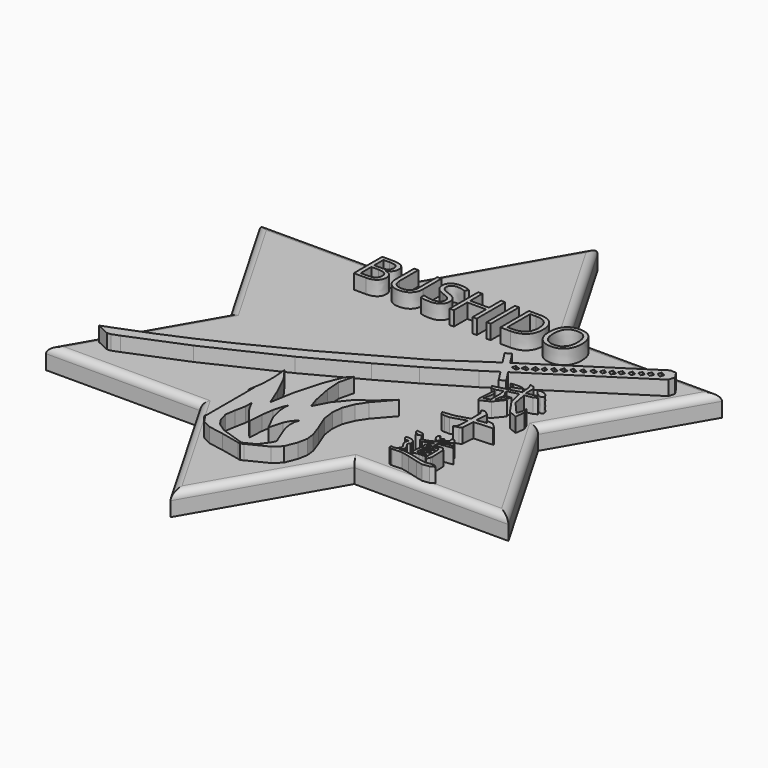
from build123d import *

# Parameters (mm, degrees)
F1_TEXT_SIZE = 8.7433378212
F5_DEPTH     = 2.54
F6_DEPTH     = 3.81
F7_R         = 1.27


# Not quite as in the source:
# - Text() gives the source's letters only with a copy of the font that has no kerning and outlines rounded to 1/6400 em; it was checked with that copy


with BuildPart() as f5:
    # F1 (on Top) + F2 (on Top) + F3 (on Top) + F4 (on Top) → F5 (new body)
    with BuildSketch(Plane.XY):
        with Locations((-18.8456885517, 15.8561766148)):
            Text('BUSHIDO', F1_TEXT_SIZE, font='Open Sans', text_align=(TextAlign.LEFT, TextAlign.BOTTOM))
    with BuildSketch(Plane.XY):
        Polygon((16.8473965077, 6.140861365), (15.3403033092, 8.4730714844), (13.8332103635, 10.8052812126), (12.9538516546, 10.2370324437), (14.4609446004, 7.9048227154), (15.9680377988, 5.5726125961), (17.3082601312, 3.4986333036), (18.2062507596, 4.0380493823), align=None)
        Polygon((33.8832835333, 20.4556965248), (15.3403033092, 8.4730714844), (16.8473965077, 6.140861365), (35.3903767318, 18.1234864055), (35.6585590299, 19.2181617838), (34.9173655604, 20.3651505113), align=None)
        Polygon((16.3403138651, 7.6048727276), (16.5452819858, 8.2522101603), (17.3955264899, 7.9045698589), (17.2131276315, 7.3285114539), align=None, mode=Mode.SUBTRACT)
        Polygon((17.5423044973, 8.2190133387), (17.6540358979, 8.9686959803), (18.5137291101, 8.6353379366), (18.4319203078, 8.0864265413), align=None, mode=Mode.SUBTRACT)
        Polygon((18.7442950032, 8.8331541453), (18.8201417398, 9.722243085), (19.6246346881, 9.4333665485), (19.567441079, 8.7629328875), align=None, mode=Mode.SUBTRACT)
        Polygon((19.880105257, 9.6755209268), (19.909781471, 10.4263771654), (20.5806503807, 10.1011195962), (20.5139143984, 9.4076129406), align=None, mode=Mode.SUBTRACT)
        Polygon((20.9012147802, 10.4437671608), (21.0185353832, 11.1428629854), (21.9333342245, 10.6891891454), (21.6664921327, 10.0982194669), align=None, mode=Mode.SUBTRACT)
        Polygon((21.9593839454, 11.1546640073), (22.1272924242, 11.8593508274), (22.9746280921, 11.5126315584), (22.8212855883, 10.9492953391), align=None, mode=Mode.SUBTRACT)
        Polygon((23.0501986545, 11.9408549982), (23.2360494653, 12.5758386693), (23.9916496211, 12.1972281915), (23.8482478404, 11.7072771993), align=None, mode=Mode.SUBTRACT)
        Polygon((24.2657142655, 12.6179341659), (24.4212694882, 13.3417375137), (25.1606684794, 12.9523679865), (25.0052522447, 12.458997356), align=None, mode=Mode.SUBTRACT)
        Polygon((25.3632898995, 13.4355934242), (25.5626688179, 14.1335176738), (26.3444185842, 13.783264237), (26.1785637478, 13.2026907586), align=None, mode=Mode.SUBTRACT)
        Polygon((26.5035142513, 14.1453166737), (26.772595353, 14.8611834628), (27.3892650859, 14.4687397575), (27.1730935281, 13.8936341928), align=None, mode=Mode.SUBTRACT)
        Polygon((27.5919822598, 14.7673956698), (27.8048862833, 15.5282582804), (28.6403827707, 15.0609908409), (28.2684432479, 14.3915536967), align=None, mode=Mode.SUBTRACT)
        Polygon((28.618680859, 15.4850552824), (28.8945260145, 16.2323923608), (29.5655970752, 15.8682429506), (29.3275818304, 15.2233970503), align=None, mode=Mode.SUBTRACT)
        Polygon((29.8286105229, 16.2127230933), (30.0606287275, 16.9859374436), (30.8057455848, 16.6156230425), (30.6141189027, 15.9770158229), align=None, mode=Mode.SUBTRACT)
        Polygon((30.8891263887, 17.0877319347), (31.2267345694, 17.7394845483), (31.8728774381, 17.2744288014), (31.5885073161, 16.7254522635), align=None, mode=Mode.SUBTRACT)
        Polygon((31.9596488099, 17.7795122535), (32.3064777484, 18.4251944804), (32.9795632278, 17.9820758951), (32.6667384259, 17.3996982665), align=None, mode=Mode.SUBTRACT)
        Polygon((33.1540412464, 18.5436265713), (33.3509214156, 19.1910772012), (34.1153814725, 18.8191470284), (33.8817490859, 18.0645479428), align=None, mode=Mode.SUBTRACT)
        Polygon((15.9680377988, 5.5726125961), (14.4609446004, 7.9048227154), (13.4392841643, 5.9546586203), align=None)
        Polygon((13.4392841643, 5.9546586203), (14.4609446004, 7.9048227154), (6.4811903646, 2.4890838609), (2.1782459322, 0.0789695365), (-3.2401958069, -2.9559439409), (-7.6722426602, -5.4383695858), (-12.9396649414, -8.1130157254), (-17.4421693546, -10.3845168919), (-23.2247509293, -13.0730367708), (-28.4219607901, -15.2921345919), (-35.5382979474, -18.067758069), (-32.8822444794, -17.7239251518), (-29.1354970118, -16.3281898003), (-23.7402903556, -14.0654356041), (-19.4283608574, -12.0606721568), (-13.5842097919, -9.1500637427), (-10.1778736561, -7.4391279445), (-6.9537364608, -5.813626828), (-3.1184731535, -3.665464522), (0.030367378, -1.9017732196), (7.4803701746, 2.4733160126), align=None)
        Polygon((13.5050336784, 3.9809992475), (15.9680377988, 5.5726125961), (13.4392841643, 5.9546586203), (7.4803701746, 2.4733160126), (0.030367378, -1.9017732196), (-3.1184731535, -3.665464522), (-6.9537364608, -5.813626828), (-10.1778736561, -7.4391279445), (-13.5842097919, -9.1500637427), (-19.4283608574, -12.0606721568), (-23.7402903556, -14.0654356041), (-29.1354970118, -16.3281898003), (-32.8822444794, -17.7239251518), (-35.5382979474, -18.067758069), (-33.2968570292, -19.1031731665), (-32.6587895882, -19.0326638095), (-31.3937997897, -18.557031558), (-21.696301016, -14.5919805452), (-8.7988901131, -8.4907568254), (0.5787971925, -3.5018383799), (6.4014223401, -0.2405384738), align=None)
    with BuildSketch(Plane.XY):
        with BuildLine():
            add(Edge.make_bspline(
                [(19.2655455321, 3.7048012018), (19.3226752676, 3.8767956934), (23.3617273428, 3.9861735046), (18.9180168874, 2.5503086332), (20.7832836423, 3.2957181778), (19.2266278514, 3.58763583), (19.2655455321, 3.7048012018)],
                knots=[0, 0, 0, 0, 0.323818666, 0.6224903435, 0.7794095959, 1, 1, 1, 1], degree=3))
        make_face()
        with BuildLine():
            add(Edge.make_bspline(
                [(23.5254075378, 4.3837185949), (23.4492975144, 4.0474977693), (25.2808853409, 2.5090790907), (25.3654259394, 4.3967328437), (23.5937132974, 4.685463593), (23.5254075378, 4.3837185949)],
                knots=[0, 0, 0, 0, 0.3876451352, 0.6521037019, 1, 1, 1, 1], degree=3))
        make_face()
        Polygon((22.2047995776, 4.9578961916), (21.5157885104, 5.1110098138), (21.8794327229, 4.5751109719), (22.0899637789, 2.6994645596), (18.3386709541, 1.7233630642), (17.573101446, 1.5511102974), (18.0515814573, 1.0152114555), (18.8171546906, 1.0152114555), (19.8698099703, 1.4362744987), (20.0420636684, 0.2496410161), (20.0420636684, -1.6642836854), (19.0468225628, -2.0470684394), (19.3530526012, -0.3245361149), (19.2190762609, 0.2305023372), (18.8171546906, 0.6898436695), (18.8171546906, 0.1348061487), (18.6492045768, -1.7791185528), (18.6492045768, -2.4860586436), (18.8554320484, -2.908334136), (20.5014068633, -2.1044863388), (21.8794327229, -0.4010936245), (21.286116913, -0.8987141773), (20.5014068633, -1.2623593211), (20.7119379193, -0.1140041277), (21.6114837676, -0.1140041277), (21.9751279801, 0.4984512925), (21.4392300695, 0.4984512925), (20.7502152771, 0.2879193053), (20.7502152771, 0.6324257702), (20.367696456, 1.0106713394), (20.2260600487, 1.5815109554), (22.1091043204, 2.0487308502), (22.7406974882, -0.496789813), (24.4058128446, -2.908334136), (25.8795339614, -3.5016518086), (26.0900687426, -1.8173977733), (25.6115850061, -0.7456000894), (25.6115850061, -1.7025619745), (25.2862181515, -2.5829672813), (23.3110389156, -0.3082971509), (22.8555332869, 2.1444270387), (24.1952817887, 2.3932373151), (24.7885975987, 2.7186041698), (24.3101175874, 3.0822493136), (22.645002231, 2.7951607481), (22.645002231, 4.5176930726), align=None)
        Polygon((21.5157885104, -4.8474837095), (21.0630316287, -4.9923323095), (21.5157885104, -5.764849484), (21.5157885104, -7.7927093953), (19.1639233381, -8.5008498281), (17.1843487769, -8.7100733072), (17.4475498688, -9.2439023334), (18.0695261806, -9.3216504902), (18.9707968384, -9.3216504902), (21.497078157, -8.5330381989), (21.497078157, -9.583117954), (21.3688183576, -10.6091815978), (20.9181848913, -11.0759101808), (21.803362295, -10.8184050769), (22.205715999, -10.576993227), (22.3666559905, -8.3720982075), (25.6659518927, -8.1628747284), (25.6659518927, -7.9214628786), (24.7456139688, -7.0922450995), (23.5254336149, -6.9397203624), (23.8810813177, -7.3615203646), (24.0726340562, -7.4386391789), (22.3505627364, -7.6800510287), (22.4954094738, -5.5395308882), (21.8799831802, -4.9941078783), align=None)
        Polygon((18.8621377283, -15.2811340253), (17.9811436683, -15.1710081846), (18.0768389255, -15.611210838), (18.6939821828, -15.9568317184), (18.5111389979, -15.9991427526), (18.5361821204, -16.2140969187), (19.3105267283, -15.8999863062), (19.2060563713, -15.4485274106), align=None)
        Polygon((21.5768984392, -14.7365058367), (21.5157885104, -14.472424984), (21.1965348572, -14.663817361), (21.1965348572, -15.0370318443), (21.4262064546, -15.4868047684), (21.9833914661, -15.8571551747), (22.4214475602, -14.769082889), (21.8759793788, -15.1135902852), align=None)
        Polygon((23.7638129647, -14.1966069276), (23.306587711, -14.1394529492), (23.3190152794, -14.1233503819), (23.2513491064, -14.2045523971), (23.2980228824, -14.407715073), (23.3731474727, -14.7323589772), (22.4867071956, -15.6797021627), (21.4378591627, -16.4037439972), (20.4228479415, -16.7217832059), (19.861208275, -16.7217832059), (19.8950450867, -16.9856846333), (20.125111565, -17.2360558063), (20.5175857991, -17.2766558826), (22.1686717123, -16.6405811906), (21.3626193817, -17.7432141374), (21.5040066593, -18.148529581), (21.407449618, -18.920974806), (21.3132735917, -20.008178609), (21.5630847961, -20.7243133336), (21.9171959752, -20.516842844), (22.4732141942, -20.4520642325), (23.216405609, -20.4520642325), (23.5897246748, -20.3656759113), (23.637091741, -20.2574077994), (23.4848428518, -19.9867356569), (23.1257693457, -19.9205675522), (22.4596802145, -20.074704662), (22.0570582896, -20.0273375958), (22.0807436854, -19.9630539864), (21.789772436, -20.0814697891), (21.8253724105, -19.4860926672), (21.8974296004, -19.3071123213), (22.8027235717, -19.3835590035), (22.4967721337, -19.6923784107), (22.5411932915, -19.753722474), (22.8912401944, -19.5002425462), (23.4110176063, -19.2575070436), (23.5028173774, -19.0294887871), (23.313710466, -18.8782345022), (22.9600204047, -18.8782345022), (22.2716163844, -19.0375354141), (21.8491461128, -19.0415587276), (21.8491461128, -18.5345932841), (22.3618656622, -18.538215652), (22.4727932364, -18.582874909), (22.283686325, -18.7438186258), (22.3520863801, -18.7920983881), (22.6225498585, -18.6044604289), (23.1688637286, -18.4138882905), (23.3901571482, -18.1925930083), (23.2131239027, -18.0195812136), (22.939523682, -17.9994627833), (22.473084689, -18.1061483228), (21.9123564241, -18.1849532703), (21.8813363463, -18.0960278958), (21.7767227441, -17.705745995), (22.0462996513, -17.5287108868), (22.4657040089, -17.5287108868), (23.1165443103, -17.613867948), (23.6008273629, -17.5018018798), (23.7630512565, -17.9668497294), (23.7630512565, -18.4846520424), (23.7630512565, -20.5501709133), (24.1183654627, -20.9745474217), (24.4008704069, -20.2728432233), (24.4458671659, -19.9128743261), (24.3618953973, -17.4610763788), (23.9151472977, -16.9732478194), (23.1065545231, -17.0868877321), (22.4024374038, -17.2920878977), (22.5030239671, -17.1472411603), (22.5554797798, -16.4739787579), (25.0591766089, -16.1221083254), (24.7107259103, -15.7783262668), (24.4122787948, -15.6581719541), (23.6246269196, -15.7499369234), (22.5589135649, -16.1216925826), (22.1833083779, -16.0747412592), (23.0562184006, -15.6890377402), (24.1033953264, -14.8758472511), (24.0441653877, -14.6198906004), align=None)
        Polygon((18.3734241873, -17.5069700927), (17.9188679904, -17.5596028566), (17.920428887, -17.6980346441), (18.030481413, -17.9564151913), (18.3223504573, -18.2291883975), (18.7054332346, -18.2291883975), (18.9330372959, -18.2633288205), (18.750956282, -18.7071599066), (18.8533756882, -19.3216931075), (19.3427298218, -20.0158897787), (19.3427298218, -20.505240187), (19.0013218671, -20.9490712732), (18.4892099351, -21.0401136428), (18.033998087, -20.9832135588), (18.033998087, -21.3359985501), (18.3412637562, -21.5522255749), (18.6712946743, -21.5522255749), (20.3669536859, -21.5067025274), (21.6984432191, -21.7912103981), (23.5534254462, -22.2919415683), (24.6800724417, -22.5536879152), (25.8750002831, -22.4057454616), (26.6260970384, -22.0074374229), (26.1822659522, -21.6774065048), (25.7156770676, -21.6774065048), (24.657310918, -21.859491244), (23.4965253621, -21.6318871826), (21.9524670392, -21.2343391031), (20.5026697367, -20.9807436913), (19.5361357182, -20.9807436913), (19.8280122131, -20.7462888211), (19.9237074703, -20.3060861677), (19.8136549443, -19.8658835143), (19.3495247513, -19.1098805517), (19.6174774319, -18.6936035752), (19.6174774319, -18.2534009218), (19.3973761052, -17.8658310324), (18.8710447401, -17.5739582628), align=None)
    with BuildSketch(Plane.XY):
        Polygon((-7.4539221823, -30.1033412686), (-7.4539221823, -29.8510509487), (-7.6599903405, -29.5398458838), align=None)
        Polygon((0.6026960909, -10.6826946139), (1.2360377375, -8.0810505897), (0.2825318837, -9.0874317454), (-1.0139159858, -12.3784067109), (-2.2429861128, -16.8394707143), (-3.0168443918, -21.1412105709), (-4.3824762106, -17.8181733936), (-5.8846697211, -14.6544594318), (-7.4551478028, -12.4922096729), (-7.2503015399, -14.9731077254), (-7.2958208621, -17.4767654389), (-7.7055096626, -20.0942270458), (-7.4539221823, -19.2088670285), (-7.4539221823, -29.8510509487), (-6.5447241068, -31.2241259962), (-4.9970075488, -32.0435035974), (-2.2657439113, -32.5214732438), (0.9336228406, -33.2185244333), (-2.7542635798, -32.2157647461), (-5.0892531872, -30.9142973274), (-6.7543685436, -28.6750048399), (-7.08600849, -27.0073313539), (-6.562974304, -25.1725222915), (-5.8356821537, -22.6461421698), (-5.6825689971, -20.3494336456), (-5.7897177957, -18.808442833), (-4.6251208991, -21.1413985735), (-3.3475793898, -24.1964217275), (-2.7741553971, -25.3451220198), (-2.1609477699, -22.0336858183), (-1.1848472059, -17.4785461277), (-0.6298087537, -15.4497865587), (0.0789985061, -13.0636664107), (-0.1350082457, -16.547055915), (0.0366674321, -19.0160583285), (0.6688386202, -21.4467030019), (1.798056066, -23.2649315149), (2.984687686, -19.8198668659), (4.1139051318, -17.8868025541), (4.7837793827, -17.1786509454), (4.2861588299, -18.9011842012), (4.2861588299, -20.9682229906), (4.6719902245, -22.908401771), (5.2813999355, -25.1597147435), (5.9321336448, -27.1884761751), (6.0852505267, -28.7387538701), (5.7981610298, -30.2698947489), (4.7837793827, -31.4756687731), (1.8726098797, -33.0832795744), (5.2717122811, -31.3864689409), (6.5788564605, -30.186602399), (7.4074827135, -28.0831716955), (7.7261291444, -26.4216531068), (7.5300708413, -24.9230805784), (6.8410560489, -22.9517370462), (5.7692602277, -20.2722419053), (5.4821707308, -18.1669257581), (5.6927017868, -16.3104180247), (6.4391344786, -14.4156320021), (7.5300708413, -12.7505175769), (10.3020183742, -9.5690198069), (8.104249835, -11.5638840944), (5.3673349321, -13.6692011729), (3.4151338041, -16.0424672067), (2.0753853023, -18.58798787), (1.4629289508, -16.7888980359), (0.7930546999, -13.4203908965), align=None)
        Polygon((-2.7542635798, -32.2157647461), (0.9336228406, -33.2185244333), (1.3987012208, -33.3198518093), (1.8726098797, -33.0832795744), (4.7837793827, -31.4756687731), (5.7981610298, -30.2698947489), (6.0852505267, -28.7387538701), (5.9321336448, -27.1884761751), (5.2813999355, -25.1597147435), (4.6719902245, -22.908401771), (4.2861588299, -20.9682229906), (4.2861588299, -18.9011842012), (4.7837793827, -17.1786509454), (4.1139051318, -17.8868025541), (2.984687686, -19.8198668659), (1.798056066, -23.2649315149), (0.6688386202, -21.4467030019), (0.0366674321, -19.0160583285), (-0.1350082457, -16.547055915), (0.0789985061, -13.0636664107), (-0.6298087537, -15.4497865587), (-1.1848472059, -17.4785461277), (-2.1609477699, -22.0336858183), (-2.7741553971, -25.3451220198), (-3.3475793898, -24.1964217275), (-4.6251208991, -21.1413985735), (-5.7897177957, -18.808442833), (-5.6825689971, -20.3494336456), (-5.8356821537, -22.6461421698), (-6.562974304, -25.1725222915), (-7.08600849, -27.0073313539), (-6.7543685436, -28.6750048399), (-5.0892531872, -30.9142973274), align=None)
        Polygon((-0.8207447827, -21.0449974984), (-0.4812404513, -20.4134136438), (-0.5489103496, -21.2524905801), (-0.4406422377, -22.4840380251), (0.0484853455, -24.3646921532), (1.4675818384, -27.1801594645), (2.1171867847, -24.8117987067), (2.6991292834, -23.6885193735), (3.592338413, -22.7817744017), (3.2727730474, -23.5929767976), (3.1998679042, -24.6764626354), (3.4705363214, -26.0433461517), (4.0879659355, -27.6435893029), (4.5707896352, -28.8989301771), (4.8922874639, -29.5429643552), (4.6273253301, -30.2155588881), (3.5024112988, -31.7638591002), (3.315448761, -32.0211891085), (1.3987012208, -32.9780174778), (-2.8003193438, -31.5866488963), (-4.3292604387, -30.5405315012), (-5.1339678466, -29.349565506), (-5.5368589181, -27.800483461), (-5.2627213299, -26.0663647205), (-4.8925541341, -24.1994448006), (-4.8925541341, -22.8314455599), (-4.1467488028, -24.3254653654), (-3.2187663019, -25.5996342748), (-1.7542019486, -27.3217055947), (-1.5987024559, -24.790639184), (-1.287471503, -22.7026920766), align=None, mode=Mode.SUBTRACT)
        Polygon((1.3987012208, -33.3198518093), (0.9336228406, -33.2185244333), (1.3987012208, -33.3449821919), (1.8726098797, -33.0832795744), align=None)
    extrude(amount=F5_DEPTH)


with BuildPart() as f6:
    # F0 (on Top) → F6 (new body)
    with BuildSketch(Plane.XY):
        Polygon((13.5116724791, -23.402903229), (40.5350174372, -23.402903229), (27.0233449582, 0), (40.5350174372, 23.402903229), (13.5116724791, 23.402903229), (0, 46.805806458), (-13.5116724791, 23.402903229), (-40.5350174372, 23.402903229), (-27.0233449582, 0), (-40.5350174372, -23.402903229), (-13.5116724791, -23.402903229), (0, -46.805806458), align=None)
    extrude(amount=-F6_DEPTH)

    # F7
    f7_edges = [f6.edges().sort_by_distance(p)[0] for p in [
        (-27.023345, -23.402903, 0),
        (-6.755836, -35.104355, 0),
        (6.755836, -35.104355, 0),
        (27.023345, -23.402903, 0),
        (33.779181, -11.701452, 0),
        (33.779181, 11.701452, 0),
        (27.023345, 23.402903, 0),
        (6.755836, 35.104355, 0),
        (-6.755836, 35.104355, 0),
        (-27.023345, 23.402903, 0),
        (-33.779181, 11.701452, 0),
        (-33.779181, -11.701452, 0),
    ]]
    fillet(f7_edges, radius=F7_R)


solid = Compound([f5.part, f6.part])
